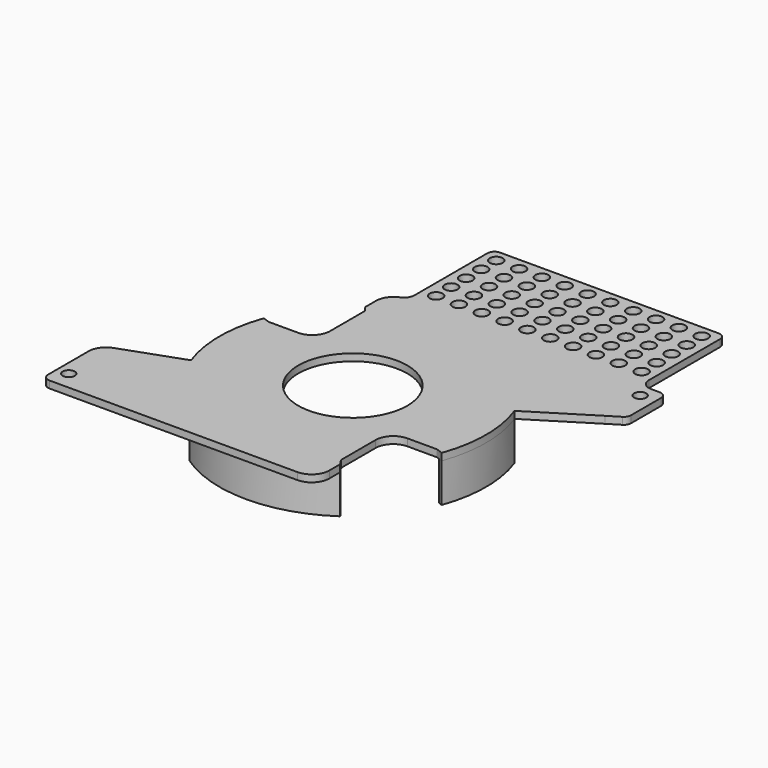
from build123d import *

# Parameters (mm, degrees)
F1_DEPTH = 11
F0_R     = 15.4518658469
F0_R_2   = 1.8318829632
F2_DEPTH = 2
F3_D     = 3.4


with BuildPart() as f1:
    # F0 (on Top) → F1 (new body)
    with BuildSketch(Plane.XY):
        with BuildLine():
            ThreePointArc((35.4919297455, -12.880666806), (37.7569682896, 0), (35.4919297455, 12.880666806))
            Line((35.4919297455, 12.880666806), (34.3639188223, 12.4712911265))
            ThreePointArc((34.3639188223, 12.4712911265), (36.5569695023, 0), (34.3639188223, -12.4712911265))
            Line((34.3639188223, -12.4712911265), (35.4919297455, -12.880666806))
        make_face()
    extrude(amount=-F1_DEPTH)


with BuildPart() as f1b:
    # F0 (on Top) → F1, piece 2 (new body)
    with BuildSketch(Plane.XY):
        with BuildLine():
            ThreePointArc((21.3512916707, 31.1401830183), (0, 37.7569682896), (-21.3512916707, 31.1401830183))
            Line((-21.3512916707, 31.1401830183), (-20.6727010615, 30.1504800959))
            ThreePointArc((-20.6727010615, 30.1504800959), (0, 36.5569695023), (20.6727010615, 30.1504800959))
            Line((20.6727010615, 30.1504800959), (21.3512916707, 31.1401830183))
        make_face()
    extrude(amount=-F1_DEPTH)


with BuildPart() as f1c:
    # F0 (on Top) → F1, piece 3 (new body)
    with BuildSketch(Plane.XY):
        with BuildLine():
            Line((21.3512916707, -31.1401830183), (20.6727010615, -30.1504800959))
            ThreePointArc((20.6727010615, -30.1504800959), (0, -36.5569695023), (-20.6727010615, -30.1504800959))
            Line((-20.6727010615, -30.1504800959), (-21.3512916707, -31.1401830183))
            ThreePointArc((-21.3512916707, -31.1401830183), (0, -37.7569682896), (21.3512916707, -31.1401830183))
        make_face()
    extrude(amount=-F1_DEPTH)


with BuildPart() as f1d:
    # F0 (on Top) → F1, piece 4 (new body)
    with BuildSketch(Plane.XY):
        with BuildLine():
            ThreePointArc((-34.3639188223, -12.4712911265), (-36.5569695023, 0), (-34.3639188223, 12.4712911265))
            Line((-34.3639188223, 12.4712911265), (-35.4919297455, 12.880666806))
            ThreePointArc((-35.4919297455, 12.880666806), (-37.7569682896, 0), (-35.4919297455, -12.880666806))
            Line((-35.4919297455, -12.880666806), (-34.3639188223, -12.4712911265))
        make_face()
    extrude(amount=-F1_DEPTH)


with BuildPart() as f2:
    # F0 (on Top) → F2 (new body)
    with BuildSketch(Plane.XY):
        with BuildLine():
            Line((54.3673303405, 39.9042378306), (52.512591213, 39.9042378306))
            ThreePointArc((52.512591213, 39.9042378306), (50.3912708694, 40.7829174871), (49.512591213, 42.9042378306))
            Line((49.512591213, 42.9042378306), (49.512591213, 68.0816214085))
            ThreePointArc((49.512591213, 68.0816214085), (48.9268047754, 69.4958349708), (47.512591213, 70.0816214085))
            Line((47.512591213, 70.0816214085), (-14.3512916707, 70.0816214085))
            ThreePointArc((-14.3512916707, 70.0816214085), (-15.7655052331, 69.4958349708), (-16.3512916707, 68.0816214085))
            Line((-16.3512916707, 68.0816214085), (-16.3512916707, 42.3204363177))
            ThreePointArc((-16.3512916707, 42.3204363177), (-16.863823078, 40.6433853346), (-18.2262916707, 39.5393618851))
            ThreePointArc((-18.2262916707, 39.5393618851), (-20.4970726587, 37.6993228025), (-21.3512916707, 34.9042378306))
            Line((-21.3512916707, 34.9042378306), (-21.3512916707, 31.1401830183))
            ThreePointArc((-21.3512916707, 31.1401830183), (0, 37.7569682896), (21.3512916707, 31.1401830183))
            Line((21.3512916707, 31.1401830183), (20.6727010615, 30.1504800959))
            ThreePointArc((20.6727010615, 30.1504800959), (0, 36.5569695023), (-20.6727010615, 30.1504800959))
            Line((-20.6727010615, 30.1504800959), (-20.2203068649, 29.4906774808))
            Line((-20.2203068649, 29.4906774808), (-20.2203068649, 17.1983737311))
            ThreePointArc((-20.2203068649, 17.1983737311), (-21.684772959, 13.6628398252), (-25.2203068649, 12.1983737311))
            Line((-25.2203068649, 12.1983737311), (-33.6119107803, 12.1983737311))
            Line((-33.6119107803, 12.1983737311), (-34.3639188223, 12.4712911265))
            ThreePointArc((-34.3639188223, 12.4712911265), (-36.5569695023, 0), (-34.3639188223, -12.4712911265))
            Line((-34.3639188223, -12.4712911265), (-35.4919297455, -12.880666806))
            Line((-35.4919297455, -12.880666806), (-52.5930077846, -18.9911596472))
            ThreePointArc((-52.5930077846, -18.9911596472), (-54.9019795203, -20.6881484667), (-55.9000037611, -23.3742365413))
            Line((-55.9000037611, -23.3742365413), (-55.9000037611, -37.9999987781))
            ThreePointArc((-55.9000037611, -37.9999987781), (-55.3142177554, -39.4142131304), (-53.9000037611, -40))
            Line((-53.9000037611, -40), (16.3512916707, -40))
            ThreePointArc((16.3512916707, -40), (19.8868255767, -38.5355339059), (21.3512916707, -35))
            Line((21.3512916707, -35), (21.3512916707, -31.1401830183))
            ThreePointArc((21.3512916707, -31.1401830183), (0, -37.7569682896), (-21.3512916707, -31.1401830183))
            Line((-21.3512916707, -31.1401830183), (-20.6727010615, -30.1504800959))
            ThreePointArc((-20.6727010615, -30.1504800959), (0, -36.5569695023), (20.6727010615, -30.1504800959))
            Line((20.6727010615, -30.1504800959), (20.2203068649, -29.4906774808))
            Line((20.2203068649, -29.4906774808), (20.2203068649, -17.1983737311))
            ThreePointArc((20.2203068649, -17.1983737311), (21.684772959, -13.6628398252), (25.2203068649, -12.1983737311))
            Line((25.2203068649, -12.1983737311), (33.6119107803, -12.1983737311))
            Line((33.6119107803, -12.1983737311), (34.3639188223, -12.4712911265))
            ThreePointArc((34.3639188223, -12.4712911265), (36.5569695023, 0), (34.3639188223, 12.4712911265))
            Line((34.3639188223, 12.4712911265), (35.4919297455, 12.880666806))
            Line((35.4919297455, 12.880666806), (52.6431709313, 23.5618650201))
            Line((52.6431709313, 23.5618650201), (55.9730917101, 25.5977149601))
            ThreePointArc((55.9730917101, 25.5977149601), (56.6743436185, 26.3259302045), (56.9298565388, 27.3040737668))
            Line((56.9298565388, 27.3040737668), (56.9298565388, 37.9042378306))
            ThreePointArc((56.9298565388, 37.9042378306), (56.3440701011, 39.318451393), (54.9298565388, 39.9042378306))
            Line((54.9298565388, 39.9042378306), (54.3673303405, 39.9042378306))
        make_face()
        Circle(F0_R, mode=Mode.SUBTRACT)
        with Locations((-12.4267879218, 45.0328276634)):
            Circle(F0_R_2, mode=Mode.SUBTRACT)
        with Locations((-5.9690505624, 45.0437702179)):
            Circle(F0_R_2, mode=Mode.SUBTRACT)
        with Locations((0.488686797, 45.0547127724)):
            Circle(F0_R_2, mode=Mode.SUBTRACT)
        with Locations((-12.4845252812, 50.4218851089)):
            Circle(F0_R_2, mode=Mode.SUBTRACT)
        with Locations((-12.5422626406, 55.8109425545)):
            Circle(F0_R_2, mode=Mode.SUBTRACT)
        with Locations((-6.0267879218, 50.4328276634)):
            Circle(F0_R_2, mode=Mode.SUBTRACT)
        with Locations((0.4309494376, 50.4437702179)):
            Circle(F0_R_2, mode=Mode.SUBTRACT)
        with Locations((-6.0845252812, 55.8218851089)):
            Circle(F0_R_2, mode=Mode.SUBTRACT)
        with Locations((0.3732120782, 55.8328276634)):
            Circle(F0_R_2, mode=Mode.SUBTRACT)
        with Locations((-12.6, 61.2)):
            Circle(F0_R_2, mode=Mode.SUBTRACT)
        with Locations((-6.1422626406, 61.2109425545)):
            Circle(F0_R_2, mode=Mode.SUBTRACT)
        with Locations((0.3154747188, 61.2218851089)):
            Circle(F0_R_2, mode=Mode.SUBTRACT)
        with Locations((-12.6577373594, 66.5890574455)):
            Circle(F0_R_2, mode=Mode.SUBTRACT)
        with Locations((-6.2, 66.6)):
            Circle(F0_R_2, mode=Mode.SUBTRACT)
        with Locations((0.2577373594, 66.6109425545)):
            Circle(F0_R_2, mode=Mode.SUBTRACT)
        with Locations((6.9464241564, 45.0656553268)):
            Circle(F0_R_2, mode=Mode.SUBTRACT)
        with Locations((13.4041615158, 45.0765978813)):
            Circle(F0_R_2, mode=Mode.SUBTRACT)
        with Locations((6.888686797, 50.4547127724)):
            Circle(F0_R_2, mode=Mode.SUBTRACT)
        with Locations((6.8309494376, 55.8437702179)):
            Circle(F0_R_2, mode=Mode.SUBTRACT)
        with Locations((13.3464241564, 50.4656553268)):
            Circle(F0_R_2, mode=Mode.SUBTRACT)
        with Locations((13.288686797, 55.8547127724)):
            Circle(F0_R_2, mode=Mode.SUBTRACT)
        with Locations((19.8618988752, 45.0875404358)):
            Circle(F0_R_2, mode=Mode.SUBTRACT)
        with Locations((26.3196362346, 45.0984829903)):
            Circle(F0_R_2, mode=Mode.SUBTRACT)
        with Locations((19.8041615158, 50.4765978813)):
            Circle(F0_R_2, mode=Mode.SUBTRACT)
        with Locations((19.7464241564, 55.8656553268)):
            Circle(F0_R_2, mode=Mode.SUBTRACT)
        with Locations((26.2618988752, 50.4875404358)):
            Circle(F0_R_2, mode=Mode.SUBTRACT)
        with Locations((26.2041615158, 55.8765978813)):
            Circle(F0_R_2, mode=Mode.SUBTRACT)
        with Locations((6.7732120782, 61.2328276634)):
            Circle(F0_R_2, mode=Mode.SUBTRACT)
        with Locations((13.2309494376, 61.2437702179)):
            Circle(F0_R_2, mode=Mode.SUBTRACT)
        with Locations((6.7154747188, 66.6218851089)):
            Circle(F0_R_2, mode=Mode.SUBTRACT)
        with Locations((13.1732120782, 66.6328276634)):
            Circle(F0_R_2, mode=Mode.SUBTRACT)
        with Locations((19.688686797, 61.2547127724)):
            Circle(F0_R_2, mode=Mode.SUBTRACT)
        with Locations((26.1464241564, 61.2656553268)):
            Circle(F0_R_2, mode=Mode.SUBTRACT)
        with Locations((19.6309494376, 66.6437702179)):
            Circle(F0_R_2, mode=Mode.SUBTRACT)
        with Locations((26.088686797, 66.6547127724)):
            Circle(F0_R_2, mode=Mode.SUBTRACT)
        with Locations((32.777373594, 45.1094255447)):
            Circle(F0_R_2, mode=Mode.SUBTRACT)
        with Locations((39.2351109535, 45.1203680992)):
            Circle(F0_R_2, mode=Mode.SUBTRACT)
        with Locations((32.7196362346, 50.4984829903)):
            Circle(F0_R_2, mode=Mode.SUBTRACT)
        with Locations((32.6618988752, 55.8875404358)):
            Circle(F0_R_2, mode=Mode.SUBTRACT)
        with Locations((39.177373594, 50.5094255447)):
            Circle(F0_R_2, mode=Mode.SUBTRACT)
        with Locations((39.1196362346, 55.8984829903)):
            Circle(F0_R_2, mode=Mode.SUBTRACT)
        with Locations((45.6928483129, 45.1313106537)):
            Circle(F0_R_2, mode=Mode.SUBTRACT)
        with Locations((45.6351109535, 50.5203680992)):
            Circle(F0_R_2, mode=Mode.SUBTRACT)
        with Locations((45.577373594, 55.9094255447)):
            Circle(F0_R_2, mode=Mode.SUBTRACT)
        with Locations((32.6041615158, 61.2765978813)):
            Circle(F0_R_2, mode=Mode.SUBTRACT)
        with Locations((39.0618988752, 61.2875404358)):
            Circle(F0_R_2, mode=Mode.SUBTRACT)
        with Locations((32.5464241564, 66.6656553268)):
            Circle(F0_R_2, mode=Mode.SUBTRACT)
        with Locations((39.0041615158, 66.6765978813)):
            Circle(F0_R_2, mode=Mode.SUBTRACT)
        with Locations((45.5196362346, 61.2984829903)):
            Circle(F0_R_2, mode=Mode.SUBTRACT)
        with Locations((45.4618988752, 66.6875404358)):
            Circle(F0_R_2, mode=Mode.SUBTRACT)
        with BuildLine():
            ThreePointArc((35.4919297455, -12.880666806), (37.7569682896, 0), (35.4919297455, 12.880666806))
            Line((35.4919297455, 12.880666806), (34.3639188223, 12.4712911265))
            ThreePointArc((34.3639188223, 12.4712911265), (36.5569695023, 0), (34.3639188223, -12.4712911265))
            Line((34.3639188223, -12.4712911265), (35.4919297455, -12.880666806))
        make_face()
        with BuildLine():
            ThreePointArc((21.3512916707, 31.1401830183), (0, 37.7569682896), (-21.3512916707, 31.1401830183))
            Line((-21.3512916707, 31.1401830183), (-20.6727010615, 30.1504800959))
            ThreePointArc((-20.6727010615, 30.1504800959), (0, 36.5569695023), (20.6727010615, 30.1504800959))
            Line((20.6727010615, 30.1504800959), (21.3512916707, 31.1401830183))
        make_face()
        with BuildLine():
            Line((21.3512916707, -31.1401830183), (20.6727010615, -30.1504800959))
            ThreePointArc((20.6727010615, -30.1504800959), (0, -36.5569695023), (-20.6727010615, -30.1504800959))
            Line((-20.6727010615, -30.1504800959), (-21.3512916707, -31.1401830183))
            ThreePointArc((-21.3512916707, -31.1401830183), (0, -37.7569682896), (21.3512916707, -31.1401830183))
        make_face()
        with BuildLine():
            ThreePointArc((-34.3639188223, -12.4712911265), (-36.5569695023, 0), (-34.3639188223, 12.4712911265))
            Line((-34.3639188223, 12.4712911265), (-35.4919297455, 12.880666806))
            ThreePointArc((-35.4919297455, 12.880666806), (-37.7569682896, 0), (-35.4919297455, -12.880666806))
            Line((-35.4919297455, -12.880666806), (-34.3639188223, -12.4712911265))
        make_face()
    extrude(amount=F2_DEPTH)

    # F3 (through all)
    with Locations(Plane(origin=(0, 0, 0), x_dir=(1, 0, 0), z_dir=(0, 0, -1))):
        with Locations((52.5918301404, -36.0042378306), (-52.6, 34.8)):
            Hole(F3_D / 2)


solid = Compound([f1.part, f1b.part, f1c.part, f1d.part, f2.part])
